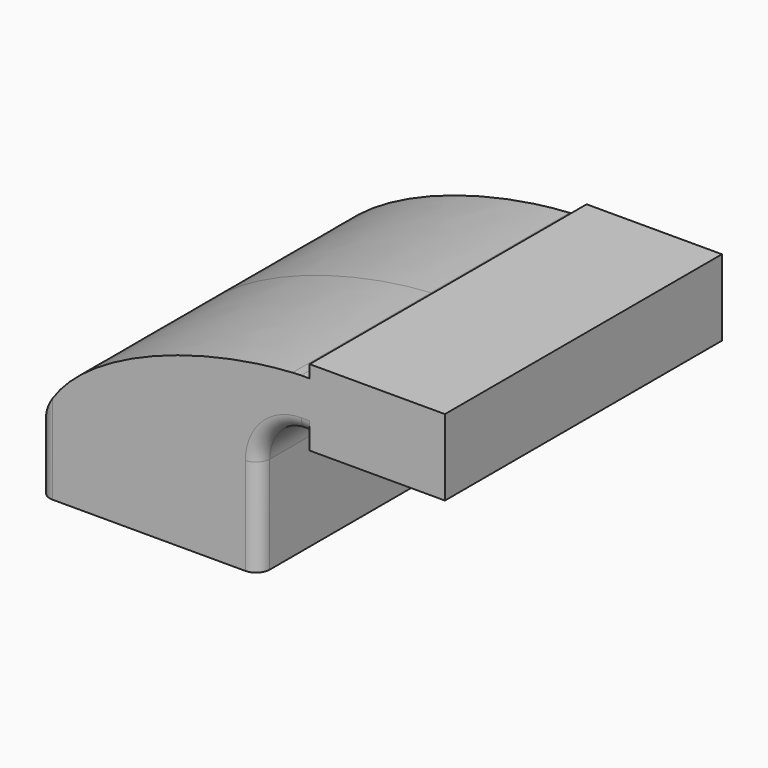
from build123d import *

# Parameters (mm, degrees)
F0_W         = 25.4
F0_H         = 19.05
F0_H_2       = 4.7498
F0_H_3       = 4.7752
F1_DEPTH     = 65
F2_DEPTH     = 25.4
F3_DEPTH     = 7.9375
F5_T1_DEPTH  = 49.2252
F5_T3_DEPTH  = 53.34
F5_T5_DEPTH  = 3.175
F5_T8_ANGLE  = 90
F5_T10_ANGLE = 90


# Not quite as in the source:
# - a fillet or chamfer that OpenCascade refuses, or shapes differently, is made with other operations: its cross-section is extruded or revolved along the edge and cut away or added


with BuildPart() as f1:
    # F0 (on Front) → F1 (new body, symmetric)
    with BuildSketch(Plane.XZ):
        Polygon((22.225, 9.525), (-41.275, 9.525), (-41.275, -9.525), (41.275, -9.525), (41.275, 9.525), align=None)
        with BuildLine():
            add(Edge.make_bspline(
                [(-41.275, 9.525), (-39.5856284224, 39.4828766469), (13.870125209, 59.4306981306), (53.8854342407, 61.7722898912)],
                knots=[0, 0, 0, 0, 108.5245810491, 108.5245810491, 108.5245810491, 108.5245810491], degree=3))
            Line((-41.275, 9.525), (22.225, 9.525))
            Line((22.225, 9.525), (22.225, 27.0002))
            ThreePointArc((22.225, 27.0002), (31.3258777096, 50.5133948686), (53.8854342407, 61.7722898912))
        make_face()
        with BuildLine():
            Line((22.225, 27.0002), (22.225, 9.525))
            Line((22.225, 9.525), (41.275, 9.525))
            Line((41.275, 9.525), (41.275, 27.0002))
            ThreePointArc((41.275, 27.0002), (45.9246798487, 38.2255201513), (57.15, 42.8752))
            Line((57.15, 42.8752), (60.325, 42.8752))
            Line((60.325, 42.8752), (60.325, 61.9252))
            Line((60.325, 61.9252), (57.15, 61.9252))
            add(Edge.make_bspline(
                [(53.8854342407, 61.7722898912), (54.9842067368, 61.8365871986), (56.0728453275, 61.8876096574), (57.15, 61.9252)],
                knots=[108.5245810491, 108.5245810491, 108.5245810491, 108.5245810491, 111.5045361635, 111.5045361635, 111.5045361635, 111.5045361635], degree=3))
            ThreePointArc((53.8854342407, 61.7722898912), (31.3258777096, 50.5133948686), (22.225, 27.0002))
        make_face()
        with Locations((73.025, 52.4002)):
            Rectangle(F0_W, F0_H)
        with Locations((73.025, 64.3001)):
            Rectangle(F0_W, F0_H_2)
        with Locations((73.025, 40.4876)):
            Rectangle(F0_W, F0_H_3)
        Polygon((85.725, 66.675), (85.725, 61.9252), (85.725, 42.8752), (85.725, 38.1), (111.125, 38.1), (111.125, 66.675), align=None)
    extrude(amount=F1_DEPTH, both=True)

    # F0 (on Front) → F2 (join, symmetric)
    with BuildSketch(Plane.XZ):
        with BuildLine():
            Line((22.225, 27.0002), (22.225, 9.525))
            Line((22.225, 9.525), (41.275, 9.525))
            Line((41.275, 9.525), (41.275, 27.0002))
            ThreePointArc((41.275, 27.0002), (45.9246798487, 38.2255201513), (57.15, 42.8752))
            Line((57.15, 42.8752), (60.325, 42.8752))
            Line((60.325, 42.8752), (60.325, 61.9252))
            Line((60.325, 61.9252), (57.15, 61.9252))
            add(Edge.make_bspline(
                [(53.8854342407, 61.7722898912), (54.9842067368, 61.8365871986), (56.0728453275, 61.8876096574), (57.15, 61.9252)],
                knots=[108.5245810491, 108.5245810491, 108.5245810491, 108.5245810491, 111.5045361635, 111.5045361635, 111.5045361635, 111.5045361635], degree=3))
            ThreePointArc((53.8854342407, 61.7722898912), (31.3258777096, 50.5133948686), (22.225, 27.0002))
        make_face()
        with Locations((73.025, 52.4002)):
            Rectangle(F0_W, F0_H)
    extrude(amount=F2_DEPTH, both=True)

    # F0 (on Front) → F3 (join, symmetric)
    with BuildSketch(Plane.XZ):
        with BuildLine():
            add(Edge.make_bspline(
                [(-41.275, 9.525), (-39.5856284224, 39.4828766469), (13.870125209, 59.4306981306), (53.8854342407, 61.7722898912)],
                knots=[0, 0, 0, 0, 108.5245810491, 108.5245810491, 108.5245810491, 108.5245810491], degree=3))
            Line((-41.275, 9.525), (22.225, 9.525))
            Line((22.225, 9.525), (22.225, 27.0002))
            ThreePointArc((22.225, 27.0002), (31.3258777096, 50.5133948686), (53.8854342407, 61.7722898912))
        make_face()
    extrude(amount=F3_DEPTH, both=True)

    # F0 (on Front) → F4 (revolve)
    with BuildSketch(Plane.XZ):
        Polygon((85.725, 66.675), (85.725, 61.9252), (85.725, 42.8752), (85.725, 38.1), (111.125, 38.1), (111.125, 66.675), align=None)
    revolve(axis=Axis((85.725, 0, 52.3875), (0, 0, 1)))

    # F5: fillet of radius 5.08 on 8 edges, made by hand

    # F5_s2 → F5_t1 (cut)
    with BuildSketch(Plane.XY.offset(-22.225)):
        with BuildLine():
            ThreePointArc((41.275, -59.92), (39.7871024484, -63.5121024484), (36.195, -65))
            Line((36.195, -65), (41.275, -65))
            Line((41.275, -65), (41.275, -59.92))
        make_face()
        with BuildLine():
            ThreePointArc((41.275, 59.92), (39.7871024484, 63.5121024484), (36.195, 65))
            Line((36.195, 65), (41.275, 65))
            Line((41.275, 65), (41.275, 59.92))
        make_face()
    extrude(amount=F5_T1_DEPTH, mode=Mode.SUBTRACT)

    # F5_s4 → F5_t3 (cut)
    with BuildSketch(Plane.XY.offset(-22.225)):
        with BuildLine():
            ThreePointArc((-41.275, -59.92), (-39.7871024484, -63.5121024484), (-36.195, -65))
            Line((-36.195, -65), (-41.275, -65))
            Line((-41.275, -65), (-41.275, -59.92))
        make_face()
        with BuildLine():
            ThreePointArc((-41.275, 59.92), (-39.7871024484, 63.5121024484), (-36.195, 65))
            Line((-36.195, 65), (-41.275, 65))
            Line((-41.275, 65), (-41.275, 59.92))
        make_face()
    extrude(amount=F5_T3_DEPTH, mode=Mode.SUBTRACT)

    # F5_s6 → F5_t5 (cut)
    with BuildSketch(Plane.YZ.offset(57.15)):
        with BuildLine():
            ThreePointArc((59.92, 42.8752), (63.5121024484, 44.3630975516), (65, 47.9552))
            Line((65, 47.9552), (65, 42.8752))
            Line((65, 42.8752), (59.92, 42.8752))
        make_face()
        with BuildLine():
            ThreePointArc((-59.92, 42.8752), (-63.5121024484, 44.3630975516), (-65, 47.9552))
            Line((-65, 47.9552), (-65, 42.8752))
            Line((-65, 42.8752), (-59.92, 42.8752))
        make_face()
    extrude(amount=F5_T5_DEPTH, mode=Mode.SUBTRACT)

    # F5_s7 → F5_t8 (revolve, cut)
    with BuildSketch(Plane.XY.offset(27.0002)):
        with BuildLine():
            ThreePointArc((41.275, 59.92), (39.7871024484, 63.5121024484), (36.195, 65))
            Line((36.195, 65), (41.275, 65))
            Line((41.275, 65), (41.275, 59.92))
        make_face()
    revolve(axis=Axis((57.15, 65, 27.0002), (0, 1, 0)), revolution_arc=F5_T8_ANGLE, mode=Mode.SUBTRACT)

    # F5_s9 → F5_t10 (revolve, cut)
    with BuildSketch(Plane.XY.offset(27.0002)):
        with BuildLine():
            ThreePointArc((41.275, -59.92), (39.7871024484, -63.5121024484), (36.195, -65))
            Line((36.195, -65), (41.275, -65))
            Line((41.275, -65), (41.275, -59.92))
        make_face()
    revolve(axis=Axis((57.15, -65, 27.0002), (0, 1, 0)), revolution_arc=F5_T10_ANGLE, mode=Mode.SUBTRACT)


solid = f1.part
